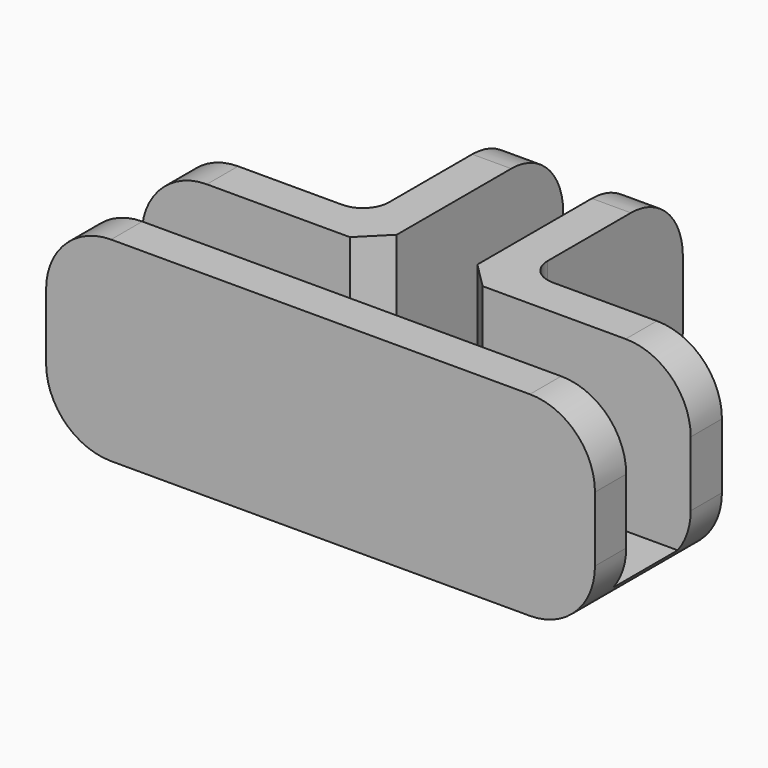
from build123d import *

# Parameters (mm, degrees)
F1_DEPTH     = 2
F2_DEPTH     = 15
F3_R         = 2
F4_T1_DEPTH  = 28
F4_T3_DEPTH  = 28
F4_T5_DEPTH  = 28
F4_T7_DEPTH  = 28
F4_T9_DEPTH  = 37.2
F4_T11_DEPTH = 37.2
F5_R         = 2
F6_SIZE      = 2


# Not quite as in the source:
# - a fillet or chamfer that OpenCascade refuses, or shapes differently, is made with other operations: its cross-section is extruded or revolved along the edge and cut away or added


with BuildPart() as f1:
    # F0 (on Top) → F1 (new body)
    with BuildSketch(Plane.XY):
        Polygon((-21.1, 0), (0, 0), (21.1, 0), (21.1, 6.2), (3.1, 6.2), (3.1, 24.2), (-3.1, 24.2), (-3.1, 6.2), (-21.1, 6.2), align=None)
        Polygon((21.1, 0), (0, 0), (-21.1, 0), (-21.1, -3), (0, -3), (21.1, -3), align=None)
        Polygon((3.1, 6.2), (21.1, 6.2), (21.1, 9.2), (6.1, 9.2), (6.1, 24.2), (3.1, 24.2), align=None)
        Polygon((-21.1, 9.2), (-21.1, 6.2), (-3.1, 6.2), (-3.1, 24.2), (-6.1, 24.2), (-6.1, 9.2), align=None)
    extrude(amount=F1_DEPTH)

    # F0 (on Top) → F2 (join)
    with BuildSketch(Plane.XY):
        Polygon((-21.1, 9.2), (-21.1, 6.2), (-3.1, 6.2), (-3.1, 24.2), (-6.1, 24.2), (-6.1, 9.2), align=None)
        Polygon((3.1, 6.2), (21.1, 6.2), (21.1, 9.2), (6.1, 9.2), (6.1, 24.2), (3.1, 24.2), align=None)
        Polygon((21.1, 0), (0, 0), (-21.1, 0), (-21.1, -3), (0, -3), (21.1, -3), align=None)
    extrude(amount=F2_DEPTH)

    # F3
    f3_edges = [f1.edges().sort_by_distance(p)[0] for p in [
        (6.1, 9.2, 7.5),
    ]]
    fillet(f3_edges, radius=F3_R)

    # F4: fillet of radius 5 on 9 edges, made by hand

    # F4_s2 → F4_t1 (cut)
    with BuildSketch(Plane.XZ.offset(-12.5)):
        with BuildLine():
            ThreePointArc((21.1, 10), (19.6355339059, 13.5355339059), (16.1, 15))
            Line((16.1, 15), (21.1, 15))
            Line((21.1, 15), (21.1, 10))
        make_face()
        with BuildLine():
            ThreePointArc((-21.1, 10), (-19.6355339059, 13.5355339059), (-16.1, 15))
            Line((-16.1, 15), (-21.1, 15))
            Line((-21.1, 15), (-21.1, 10))
        make_face()
    extrude(amount=F4_T1_DEPTH, mode=Mode.SUBTRACT)

    # F4_s4 → F4_t3 (cut)
    with BuildSketch(Plane.XZ.offset(-21.7)):
        with BuildLine():
            ThreePointArc((21.1, 10), (19.6355339059, 13.5355339059), (16.1, 15))
            Line((16.1, 15), (21.1, 15))
            Line((21.1, 15), (21.1, 10))
        make_face()
        with BuildLine():
            ThreePointArc((-21.1, 10), (-19.6355339059, 13.5355339059), (-16.1, 15))
            Line((-16.1, 15), (-21.1, 15))
            Line((-21.1, 15), (-21.1, 10))
        make_face()
    extrude(amount=F4_T3_DEPTH, mode=Mode.SUBTRACT)

    # F4_s6 → F4_t5 (cut)
    with BuildSketch(Plane.YZ.offset(-18.6)):
        with BuildLine():
            ThreePointArc((24.2, 10), (22.7355339059, 13.5355339059), (19.2, 15))
            Line((19.2, 15), (24.2, 15))
            Line((24.2, 15), (24.2, 10))
        make_face()
    extrude(amount=F4_T5_DEPTH, mode=Mode.SUBTRACT)

    # F4_s8 → F4_t7 (cut)
    with BuildSketch(Plane.YZ.offset(-9.4)):
        with BuildLine():
            ThreePointArc((24.2, 10), (22.7355339059, 13.5355339059), (19.2, 15))
            Line((19.2, 15), (24.2, 15))
            Line((24.2, 15), (24.2, 10))
        make_face()
    extrude(amount=F4_T7_DEPTH, mode=Mode.SUBTRACT)

    # F4_s10 → F4_t9 (cut)
    with BuildSketch(Plane.XZ.offset(-21.7)):
        with BuildLine():
            ThreePointArc((-16.1, 0), (-19.6355339059, 1.4644660941), (-21.1, 5))
            Line((-21.1, 5), (-21.1, 0))
            Line((-21.1, 0), (-16.1, 0))
        make_face()
        with BuildLine():
            ThreePointArc((16.1, 0), (19.6355339059, 1.4644660941), (21.1, 5))
            Line((21.1, 5), (21.1, 0))
            Line((21.1, 0), (16.1, 0))
        make_face()
    extrude(amount=F4_T9_DEPTH, mode=Mode.SUBTRACT)

    # F4_s12 → F4_t11 (cut)
    with BuildSketch(Plane.YZ.offset(-18.6)):
        with BuildLine():
            ThreePointArc((19.2, 0), (22.7355339059, 1.4644660941), (24.2, 5))
            Line((24.2, 5), (24.2, 0))
            Line((24.2, 0), (19.2, 0))
        make_face()
    extrude(amount=F4_T11_DEPTH, mode=Mode.SUBTRACT)

    # F5
    f5_edges = [f1.edges().sort_by_distance(p)[0] for p in [
        (-6.1, 9.2, 7.5),
    ]]
    fillet(f5_edges, radius=F5_R)

    # F6
    f6_edges = [f1.edges().sort_by_distance(p)[0] for p in [
        (3.1, 6.2, 8.5),
        (-3.1, 6.2, 8.5),
    ]]
    chamfer(f6_edges, length=F6_SIZE)


solid = f1.part
